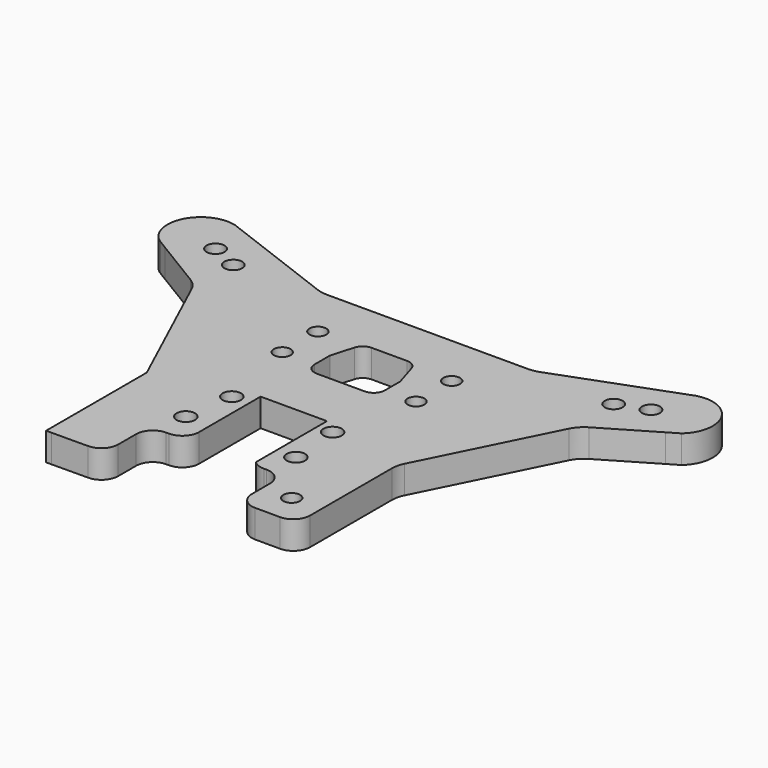
from build123d import *

# Parameters (mm, degrees)
F0_R      = 1.5
F0_R_2    = 1.6
F1_DEPTH  = 5
F2_R      = 3
F3_R      = 2
F4_R      = 5
F5_R      = 5
F6_R      = 1.5
F7_DEPTH  = 25
F9_DEPTH  = 25
F10_R     = 2
F11_R     = 1.65
F12_DEPTH = 25
F14_DEPTH = 25


with BuildPart() as f1:
    # F0 (on Top) → F1 (new body)
    with BuildSketch(Plane.XY):
        with BuildLine():
            Line((-9.9999813339, 0.0193215341), (0, 0))
            Line((0, 0), (0.4539924878, 0))
            Line((0.4539924878, 0), (0.4539924878, 22.4998891728))
            Line((0.4539924878, 22.4998891728), (12.9539924878, 47.5548288056))
            Line((12.9539924878, 47.5548288056), (23.5864712774, 53.8304637924))
            Line((23.5864712774, 53.8304637924), (25.5346026442, 54.9803143218))
            ThreePointArc((25.5346026442, 54.9803143218), (26.8013490925, 62.2870919693), (19.9533457596, 65.1328777146))
            Line((19.9533457596, 65.1328777146), (19.1141014773, 64.8209017638))
            Line((19.1141014773, 64.8209017638), (-2.4981679914, 56.7868782273))
            Line((-2.4981679914, 56.7868782273), (-40.5460603337, 56.7868782273))
            Line((-40.5460603337, 56.7868782273), (-61.6849283551, 64.8209017638))
            Line((-61.6849283551, 64.8209017638), (-62.7787610133, 65.2366230461))
            ThreePointArc((-62.7787610133, 65.2366230461), (-69.534777582, 62.3971715251), (-68.4220804384, 55.1536813523))
            Line((-68.4220804384, 55.1536813523), (-66.3019318016, 53.8657127229))
            Line((-66.3019318016, 53.8657127229), (-56.0460603337, 47.6353756185))
            Line((-56.0460603337, 47.6353756185), (-44.4999813339, 22.5804359857))
            Line((-44.4999813339, 22.5804359857), (-44.4999813339, 0))
            Line((-44.4999813339, 0), (-43.5460603337, 0))
            Line((-43.5460603337, 0), (-33.9999813339, 0.0656933026))
            Line((-33.9999813339, 0.0656933026), (-33.9999813339, 10.0656933026))
            Line((-33.9999813339, 10.0656933026), (-27.4999813339, 10.0656933026))
            Line((-27.4999813339, 10.0656933026), (-27.4999813339, 22.5656933026))
            Line((-27.4999813339, 22.5656933026), (-27.4999813339, 26.3816152201))
            Line((-27.4999813339, 26.3816152201), (-16.4999813339, 26.3816152201))
            Line((-16.4999813339, 26.3816152201), (-16.4999813339, 10.0656933026))
            Line((-16.4999813339, 10.0656933026), (-9.9999813339, 10.0656933026))
            Line((-9.9999813339, 10.0656933026), (-9.9999813339, 0.0193215341))
        make_face()
        with Locations((-4.888762403, 5.563379294)):
            Circle(F0_R, mode=Mode.SUBTRACT)
        with Locations((-55.4315750417, 55.6511066578)):
            Circle(F0_R_2, mode=Mode.SUBTRACT)
        with Locations((-60.4380198654, 57.9282781987)):
            Circle(F0_R_2, mode=Mode.SUBTRACT)
        with Locations((12.5329179775, 55.9733003324)):
            Circle(F0_R_2, mode=Mode.SUBTRACT)
        with Locations((17.6882422101, 57.8897115767)):
            Circle(F0_R_2, mode=Mode.SUBTRACT)
    extrude(amount=F1_DEPTH)

    # F2
    f2_edges = [f1.edges().sort_by_distance(p)[0] for p in [
        (-27.499981, 10.065693, 2.5),
        (-33.999981, 10.065693, 2.5),
        (-16.499981, 10.065693, 2.5),
        (-9.999981, 10.065693, 2.5),
        (-9.999981, 0.019322, 2.5),
        (-33.999981, 0.065693, 2.5),
        (-43.54606, 0, 2.5),
        (0.453992, 0, 2.5),
    ]]
    fillet(f2_edges, radius=F2_R)

    # F3
    f3_edges = [f1.edges().sort_by_distance(p)[0] for p in [
        (-16.499981, 26.381615, 2.5),
    ]]
    fillet(f3_edges, radius=F3_R)

    # F4
    f4_edges = [f1.edges().sort_by_distance(p)[0] for p in [
        (-43.54606, 0, 2.5),
        (0.453992, 22.499889, 2.5),
    ]]
    fillet(f4_edges, radius=F4_R)

    # F5
    f5_edges = [f1.edges().sort_by_distance(p)[0] for p in [
        (12.953992, 47.554829, 2.5),
        (-2.498168, 56.786878, 2.5),
        (-40.54606, 56.786878, 2.5),
        (-68.42208, 55.153681, 2.5),
        (-56.04606, 47.635376, 2.5),
    ]]
    fillet(f5_edges, radius=F5_R)

    # F6 (on face) → F7 (cut)
    with BuildSketch(Plane.XY.offset(5)):
        with Locations((-33.5573396883, 47.271139662)):
            Circle(F6_R)
        with Locations((-33.5573396883, 39.271139662)):
            Circle(F6_R)
        with Locations((-9.5573396883, 39.271139662)):
            Circle(F6_R)
        with Locations((-9.5573396883, 47.271139662)):
            Circle(F6_R)
    extrude(amount=-F7_DEPTH, mode=Mode.SUBTRACT)

    # F8 (on face) → F9 (cut)
    with BuildSketch(Plane.XY.offset(5)):
        Polygon((-16.7706497014, 48.1220260262), (-26.0973814875, 48.1220260262), (-27.693849057, 42.6604263484), (-27.693849057, 37.1988266706), (-15.0901572779, 37.1988266706), (-15.0901572779, 42.6604263484), align=None)
    extrude(amount=-F9_DEPTH, mode=Mode.SUBTRACT)

    # F10
    f10_edges = [f1.edges().sort_by_distance(p)[0] for p in [
        (-26.097381, 48.122026, 2.5),
        (-16.77065, 48.122026, 2.5),
        (-27.693849, 37.198827, 2.5),
        (-15.090157, 37.198827, 2.5),
    ]]
    fillet(f10_edges, radius=F10_R)

    # F11 (on face) → F12 (cut)
    with BuildSketch(Plane.XY.offset(5)):
        with Locations((-31.8884050022, 15.5689349914)):
            Circle(F11_R)
        with Locations((-12.1384050022, 15.5689349914)):
            Circle(F11_R)
        with Locations((-30.6362952974, 24.3189349914)):
            Circle(F11_R)
        with BuildLine():
            ThreePointArc((-11.241093269, 24.7316152201), (-13.0990926805, 26.368452489), (-14.4886523536, 24.3189349914))
            Line((-14.4886523536, 24.3189349914), (-11.2935341844, 24.3189349914))
            ThreePointArc((-11.2935341844, 24.3189349914), (-11.2542560001, 24.5236158086), (-11.241093269, 24.7316152201))
        make_face()
        with BuildLine():
            Line((-11.2935341844, 24.3189349914), (-14.4886523536, 24.3189349914))
            ThreePointArc((-14.4886523536, 24.3189349914), (-12.891093269, 23.0816152201), (-11.2935341844, 24.3189349914))
        make_face()
    extrude(amount=-F12_DEPTH, mode=Mode.SUBTRACT)

    # F13 (on face) → F14 (cut)
    with BuildSketch(Plane.XY.offset(5)):
        Polygon((-27.4999813339, 26.8493555486), (-27.4999813339, 24.3816152201), (-15.5926216394, 8.9839491993), (-15.5926216394, 26.8493555486), (-16.1031354219, 26.8493555486), align=None)
    extrude(amount=-F14_DEPTH, mode=Mode.SUBTRACT)


solid = f1.part
